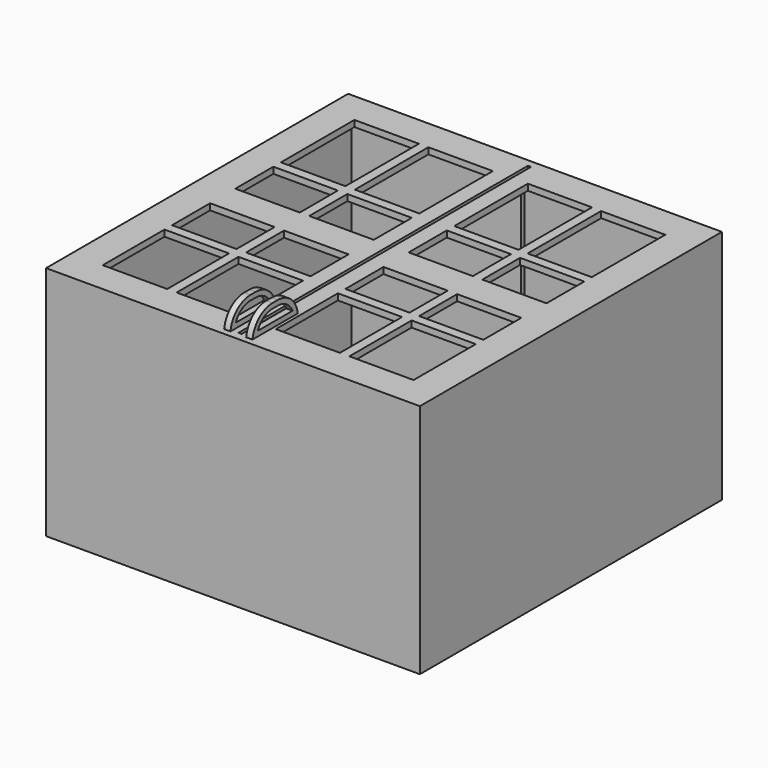
from build123d import *

# Parameters (mm, degrees)
F0_W           = 594
F0_H           = 600
F1_DEPTH       = 365
F2_W           = 544.0000259457
F2_H           = 550.0000259457
F3_DEPTH       = 360
F4_W           = 594
F4_H           = 600
F4_W_2         = 544.0000259457
F4_H_2         = 550.0000259457
F5_DEPTH       = 10
F6_W           = 102.5
F6_H           = 146
F6_H_2         = 75.6546143503
F6_W_2         = 102
F6_H_3         = 74.9739574221
F6_H_4         = 75.5056260526
F6_H_5         = 123.5204165253
F6_H_6         = 123.3714282276
F6_H_7         = 122.8397595971
F6_H_8         = 122.6907712994
F7_DEPTH       = 350
F8_W           = 10
F8_H           = 90
F9_DEPTH       = 35
F10_T1_DEPTH   = 208.4313483298
F10_2_T1_DEPTH = 208.4313483298
F12_DEPTH      = 100


# Not quite as in the source:
# - a fillet or chamfer that OpenCascade refuses, or shapes differently, is made with other operations: its cross-section is extruded or revolved along the edge and cut away or added


with BuildPart() as f1:
    # F0 (on Top) → F1 (new body)
    with BuildSketch(Plane.XY):
        with Locations((-2.3632310331, 36.6546143503)):
            Rectangle(F0_W, F0_H)
    extrude(amount=F1_DEPTH)

    # F2 (on face) → F3 (cut)
    with BuildSketch(Plane.XY.offset(365)):
        with Locations((-2.3632310331, 36.6546143503)):
            Rectangle(F2_W, F2_H)
    extrude(amount=-F3_DEPTH, mode=Mode.SUBTRACT)

    # F4 (on face) → F5 (join)
    with BuildSketch(Plane.XY.offset(365)):
        with Locations((-2.3632310331, 36.6546143503)):
            Rectangle(F4_W, F4_H)
        with Locations((-2.3632310331, 36.6546143503)):
            Rectangle(F4_W_2, F4_H_2, mode=Mode.SUBTRACT)
        with Locations((-2.3632310331, 36.6546143503)):
            Rectangle(F4_W_2, F4_H_2)
    extrude(amount=F5_DEPTH)

    # F6 (on face) → F7 (cut)
    with BuildSketch(Plane.XY.offset(375)):
        with Locations((-198.1132310331, 213.6546143503)):
            Rectangle(F6_W, F6_H)
        with Locations((-80.6132310331, 213.6546143503)):
            Rectangle(F6_W, F6_H)
        with Locations((-80.6132310331, 87.8273071751)):
            Rectangle(F6_W, F6_H_2)
        with Locations((-198.1132310331, 87.8273071751)):
            Rectangle(F6_W, F6_H_2)
        with Locations((76.6367689669, 214.3352712785)):
            Rectangle(F6_W_2, F6_H)
        with Locations((193.6367689669, 213.6546143503)):
            Rectangle(F6_W_2, F6_H)
        with Locations((193.6367689669, 88.1676356392)):
            Rectangle(F6_W_2, F6_H_3)
        with Locations((76.6367689669, 88.5079641033)):
            Rectangle(F6_W_2, F6_H_2)
        with Locations((76.6367689669, -37.146650247)):
            Rectangle(F6_W_2, F6_H_2)
        with Locations((193.6367689669, -37.0721560981)):
            Rectangle(F6_W_2, F6_H_4)
        with Locations((193.6367689669, -151.5851773871)):
            Rectangle(F6_W_2, F6_H_5)
        with Locations((76.6367689669, -151.6596715359)):
            Rectangle(F6_W_2, F6_H_6)
        with Locations((-80.6132310331, -151.9255058512)):
            Rectangle(F6_W, F6_H_7)
        with Locations((-80.6132310331, -37.7528130263)):
            Rectangle(F6_W, F6_H_4)
        with Locations((-198.1132310331, -37.8273071751)):
            Rectangle(F6_W, F6_H_2)
        with Locations((-198.1132310331, -152)):
            Rectangle(F6_W, F6_H_8)
        Polygon((0.6367689669, -249.8852461576), (0.6367689669, 324.9841928482), (-4.3632310331, 324.9841928482), (-4.3632310331, -249.8852461576), (0, -249.8852461576), align=None)
    extrude(amount=-F7_DEPTH, mode=Mode.SUBTRACT)


with BuildPart() as f9:
    # F8 (on face) → F9 (new body)
    with BuildSketch(Plane.XY.offset(375)):
        with Locations((-19.3632310331, -208.3453856497)):
            Rectangle(F8_W, F8_H)
    extrude(amount=F9_DEPTH)

    # F10: fillet of radius 40 on 2 edges, made by hand

    # F10_s2 → F10_t1 (cut)
    with BuildSketch(Plane.YZ.offset(-123.578905198)):
        with BuildLine():
            ThreePointArc((-163.3453856497, 375), (-176.574142205, 400), (-203.0316553157, 410))
            Line((-203.0316553157, 410), (-163.3453856497, 410))
            Line((-163.3453856497, 410), (-163.3453856497, 375))
        make_face()
        with BuildLine():
            ThreePointArc((-253.3453856497, 375), (-240.1166290944, 400), (-213.6591159837, 410))
            Line((-213.6591159837, 410), (-253.3453856497, 410))
            Line((-253.3453856497, 410), (-253.3453856497, 375))
        make_face()
    extrude(amount=F10_T1_DEPTH, mode=Mode.SUBTRACT)


with BuildPart() as f9b:
    # F8 (on face) → F9, piece 2 (new body)
    with BuildSketch(Plane.XY.offset(375)):
        with Locations((15.6367689669, -208.3453856497)):
            Rectangle(F8_W, F8_H)
    extrude(amount=F9_DEPTH)

    # F10#2: fillet of radius 40 on 2 edges, made by hand

    # F10_2_s2 → F10_2_t1 (cut)
    with BuildSketch(Plane.YZ.offset(-88.578905198)):
        with BuildLine():
            ThreePointArc((-163.3453856497, 375), (-176.574142205, 400), (-203.0316553157, 410))
            Line((-203.0316553157, 410), (-163.3453856497, 410))
            Line((-163.3453856497, 410), (-163.3453856497, 375))
        make_face()
        with BuildLine():
            ThreePointArc((-253.3453856497, 375), (-240.1166290944, 400), (-213.6591159837, 410))
            Line((-213.6591159837, 410), (-253.3453856497, 410))
            Line((-253.3453856497, 410), (-253.3453856497, 375))
        make_face()
    extrude(amount=F10_2_T1_DEPTH, mode=Mode.SUBTRACT)


with BuildPart() as f12_tool:
    # F11 (on face) → F12 (new body)
    with BuildSketch(Plane(origin=(-24.3632310331, 0, 0), x_dir=(0, -1, 0), z_dir=(-1, 0, 0))):
        with BuildLine():
            ThreePointArc((242.8995144287, 382.9999899864), (231.094723675, 396.8328199283), (213.6591159837, 402.0000100136))
            Line((213.6591159837, 402.0000100136), (203.0316553157, 402.0000100136))
            ThreePointArc((203.0316553157, 402.0000100136), (185.5960476244, 396.8328199283), (173.7912568707, 382.9999899864))
            Line((173.7912568707, 382.9999899864), (242.8995144287, 382.9999899864))
        make_face()
    extrude(amount=-F12_DEPTH)


with BuildPart() as f9_1:
    add(f9.part)

    # F12: cut by f12_tool
    add(f12_tool.part, mode=Mode.SUBTRACT)


with BuildPart() as f9b_1:
    add(f9b.part)

    # F12: cut by f12_tool
    add(f12_tool.part, mode=Mode.SUBTRACT)


solid = Compound([f1.part, f9_1.part, f9b_1.part])
